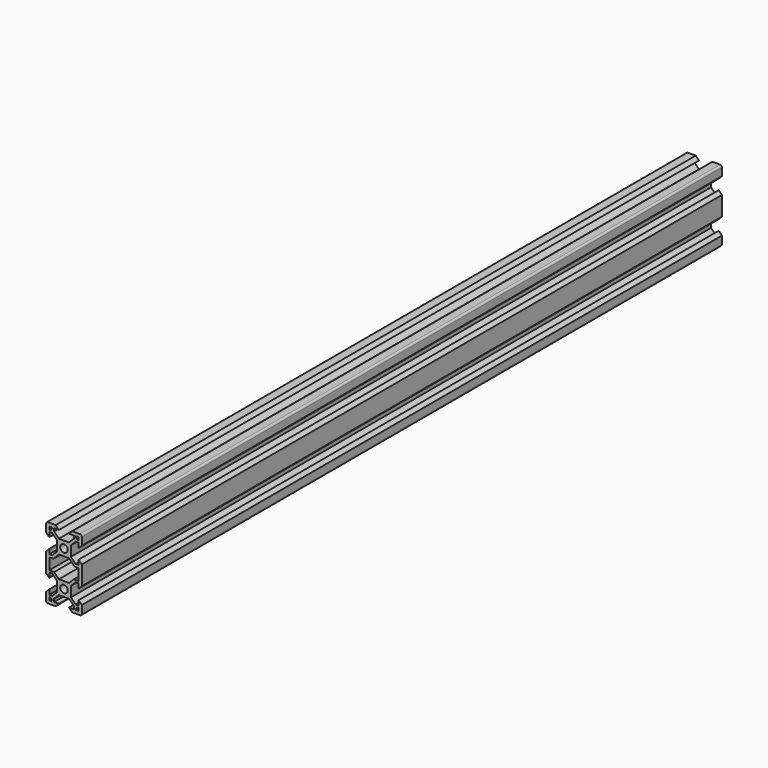
from build123d import *

# Parameters (mm, degrees)
F0_W             = 20
F0_H             = 20
F1_DEPTH         = 448
F2_R             = 2.1
F3_DEPTH         = 448.001
F4_R             = 1
F6_DEPTH         = 448.001
F6_COPIES3_COUNT = 2
F6_COPIES3_ANGLE = 90
F6_COPIES4_COUNT = 2
F6_COPIES4_ANGLE = 270
F6_COPIES6_COUNT = 2
F9_W             = 16.4
F9_H             = 6.8613203436
F10_DEPTH        = 448.001
F12_DEPTH        = 448


# Not quite as in the source:
# - a pattern or mirror of a feature is missing from the dataset's text; its kind, count and spacing are read off the source's solid


with BuildPart() as f1:
    # F0 (on Front) → F1 (new body)
    with BuildSketch(Plane.XZ):
        Rectangle(F0_W, F0_H)
    extrude(amount=F1_DEPTH)

    # F2 (on face) → F3 (cut, through all)
    with BuildSketch(Plane.XZ.offset(448)):
        Circle(F2_R)
    extrude(amount=-F3_DEPTH, mode=Mode.SUBTRACT)

    # F4
    f4_edges = [f1.edges().sort_by_distance(p)[0] for p in [
        (-10, -224, 10),
        (10, -224, 10),
    ]]
    fillet(f4_edges, radius=F4_R)

    # F5 (on face) → F6 (cut, through all)
    with BuildSketch(Plane.XZ.offset(448)):
        Polygon((0, 3.9006601718), (0, 10), (-2.84, 10), (-4.64, 10), (-2.84, 8.2), (-5.4993398282, 8.2), (-5.4993398282, 6.56), (-2.84, 3.9006601718), align=None)
        Polygon((-6.5693398282, 8.2), (-8.2, 8.2), (-7.0953059148, 7.0953059148), (-6.5693398282, 7.6212720014), align=None)
    f6 = extrude(amount=-F6_DEPTH, mode=Mode.SUBTRACT)

    # F6_copies: F6 across plane
    add(f6.mirror(Plane(origin=(0, 0, 0), x_dir=(-0.7071067812, 0, -0.7071067812), z_dir=(0.7071067812, 0, -0.7071067812))), mode=Mode.SUBTRACT)

    # F6_copies1: F6 across plane
    add(f6.mirror(Plane(origin=(0, 0, 0), x_dir=(0.7071067812, 0, -0.7071067812), z_dir=(-0.7071067812, 0, -0.7071067812))), mode=Mode.SUBTRACT)

    # F6_copies2: F6 across plane
    add(f6.mirror(Plane(origin=(0, 0, 0), x_dir=(0, 0, 1), z_dir=(1, 0, 0))), mode=Mode.SUBTRACT)

    # F6_copies3: F6 ×2 about axis
    f6_copies3_axis = Axis((0, 0, 0), (0, 1, 0))
    for i in range(1, F6_COPIES3_COUNT):
        add(f6.rotate(f6_copies3_axis, i * F6_COPIES3_ANGLE / (F6_COPIES3_COUNT - 1)), mode=Mode.SUBTRACT)

    # F6_copies4: F6 ×2 about axis
    f6_copies4_axis = Axis((0, 0, 0), (0, 1, 0))
    for i in range(1, F6_COPIES4_COUNT):
        add(f6.rotate(f6_copies4_axis, i * F6_COPIES4_ANGLE / (F6_COPIES4_COUNT - 1)), mode=Mode.SUBTRACT)

    # F6_copies5: F6 across plane
    add(f6.mirror(Plane(origin=(0, 0, 0), x_dir=(-1, 0, 0), z_dir=(0, 0, -1))), mode=Mode.SUBTRACT)

    # F6_copies6: F6 ×2 about axis
    f6_copies6_axis = Axis((0, 0, 0), (0, 1, 0))
    for i in range(1, F6_COPIES6_COUNT):
        add(f6.rotate(f6_copies6_axis, i * 360 / F6_COPIES6_COUNT), mode=Mode.SUBTRACT)

    # F8: F1 across face


with BuildPart() as f1_1:
    add(f1.part)
    add(f1.part.mirror(Plane(origin=(-7.32, -224, -10), x_dir=(1, 0, 0), z_dir=(0, 0, -1))))

    # F9 (on face) → F10 (cut, through all)
    with BuildSketch(Plane.XZ.offset(448)):
        with Locations((0, -10)):
            Rectangle(F9_W, F9_H)
    extrude(amount=-F10_DEPTH, mode=Mode.SUBTRACT)

    # F11 (on face) → F12 (join, through all)
    with BuildSketch(Plane.XZ.offset(448)):
        with BuildLine():
            ThreePointArc((-9, -10), (-9.7071067812, -9.7071067812), (-10, -9))
            Line((-10, -9), (-10, -11))
            ThreePointArc((-10, -11), (-9.7071067812, -10.2928932188), (-9, -10))
        make_face()
        with BuildLine():
            ThreePointArc((10, -9), (9.7071067812, -9.7071067812), (9, -10))
            ThreePointArc((9, -10), (9.7071067812, -10.2928932188), (10, -11))
            Line((10, -11), (10, -9))
        make_face()
        Polygon((5.9386796564, -6.9993398282), (8.2, -6.9993398282), (8.2, -6.5693398282), (5.5086796564, -6.5693398282), align=None)
        Polygon((-8.2, -6.5693398282), (-8.2, -6.9993398282), (-5.9386796564, -6.9993398282), (-5.5086796564, -6.5693398282), align=None)
    extrude(amount=-F12_DEPTH)


solid = f1_1.part
